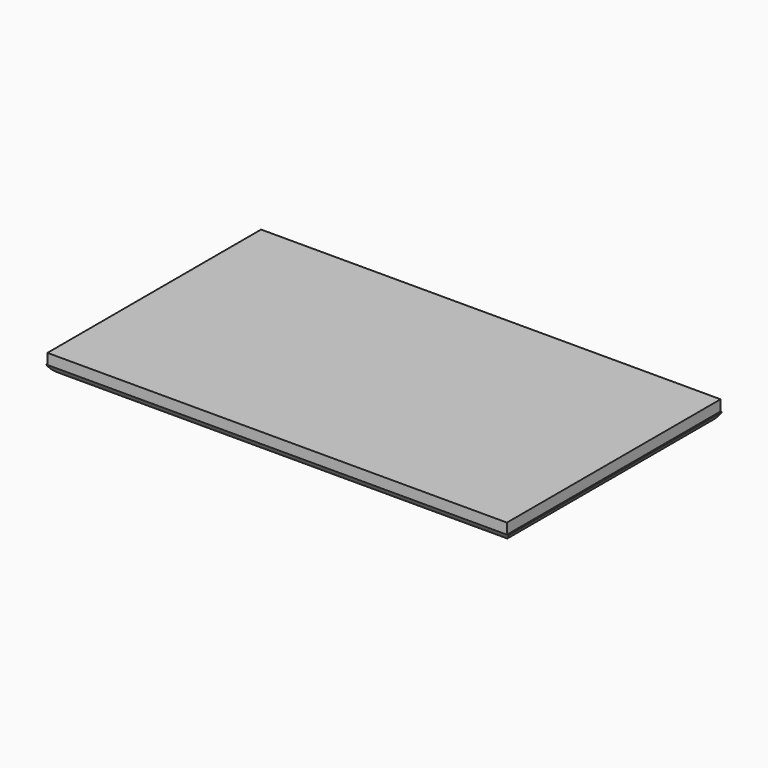
from build123d import *

# Parameters (mm, degrees)
F0_W        = 130
F0_H        = 75
F1_DEPTH    = 3
F2_T1_DEPTH = 153.1732604525
F2_T3_DEPTH = 98.1732604525
F4_W        = 129.1797161102
F4_H        = 75.0736519694
F5_DEPTH    = 3


# Not quite as in the source:
# - a fillet or chamfer that OpenCascade refuses, or shapes differently, is made with other operations: its cross-section is extruded or revolved along the edge and cut away or added


with BuildPart() as f1:
    # F0 (on Top) → F1 (new body)
    with BuildSketch(Plane.XY):
        Rectangle(F0_W, F0_H)
    extrude(amount=F1_DEPTH)

    # F2: fillet of radius 5.08 on 4 edges, made by hand

    # F2_s2 → F2_t1 (cut)
    with BuildSketch(Plane.YZ.offset(-76.5866302263)):
        with BuildLine():
            ThreePointArc((37.5, 3), (35.6257826579, 0.8154484409), (32.8653479095, 0))
            Line((32.8653479095, 0), (37.5, 0))
            Line((37.5, 0), (37.5, 3))
        make_face()
        with BuildLine():
            ThreePointArc((-37.5, 3), (-35.6257826579, 0.8154484409), (-32.8653479095, 0))
            Line((-32.8653479095, 0), (-37.5, 0))
            Line((-37.5, 0), (-37.5, 3))
        make_face()
    extrude(amount=F2_T1_DEPTH, mode=Mode.SUBTRACT)

    # F2_s4 → F2_t3 (cut)
    with BuildSketch(Plane.XZ.offset(-49.0866302263)):
        with BuildLine():
            ThreePointArc((65, 3), (63.1257826579, 0.8154484409), (60.3653479095, 0))
            Line((60.3653479095, 0), (65, 0))
            Line((65, 0), (65, 3))
        make_face()
        with BuildLine():
            ThreePointArc((-65, 3), (-63.1257826579, 0.8154484409), (-60.3653479095, 0))
            Line((-60.3653479095, 0), (-65, 0))
            Line((-65, 0), (-65, 3))
        make_face()
    extrude(amount=F2_T3_DEPTH, mode=Mode.SUBTRACT)

    # F4 (on face) → F5 (join)
    with BuildSketch(Plane.XY.offset(3)):
        Rectangle(F4_W, F4_H)
    extrude(amount=F5_DEPTH)


solid = f1.part
